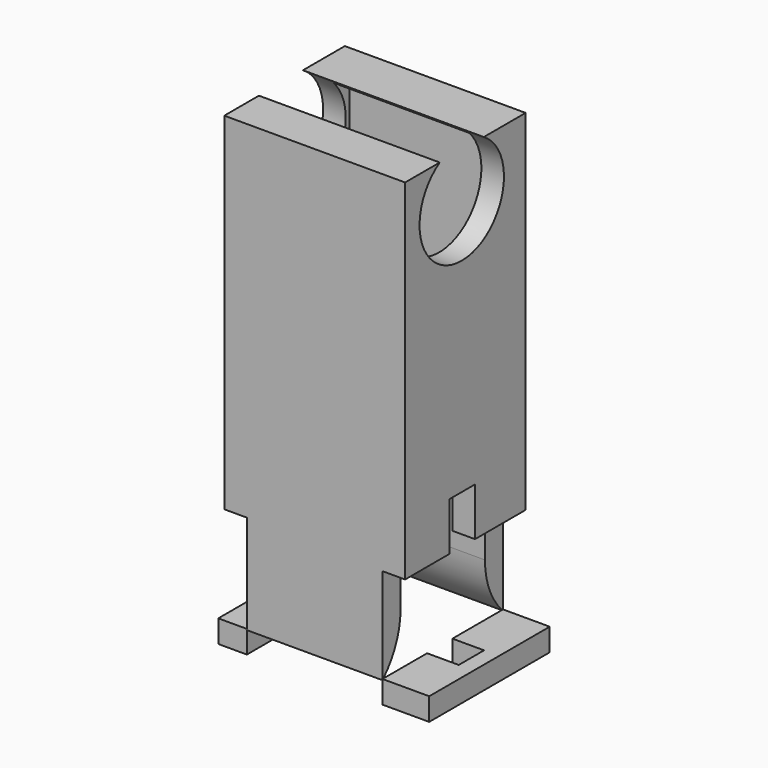
from build123d import *

# Parameters (mm, degrees)
F0_W         = 14
F0_H         = 10
F1_DEPTH     = 1.5
F2_W         = 9
F2_H         = 7
F3_DEPTH     = 25
F4_W         = 12
F4_H         = 10
F4_W_2       = 9
F4_H_2       = 7
F5_DEPTH     = 29
F6_W         = 12
F6_H         = 10
F7_DEPTH     = 0.5
F8_R         = 3.5
F9_DEPTH     = 25
F10_W        = 2.1
F10_H        = 2.1
F11_DEPTH    = 11
F12_W        = 10
F12_H        = 6.5
F13_DEPTH    = 1.5
F14_W        = 10
F14_H        = 6.3
F15_DEPTH    = 1.5
F16_T1_DEPTH = 9


# Not quite as in the source:
# - a fillet or chamfer that OpenCascade refuses, or shapes differently, is made with other operations: its cross-section is extruded or revolved along the edge and cut away or added


with BuildPart() as f1:
    # F0 (on Top) → F1 (new body)
    with BuildSketch(Plane.XY):
        with Locations((7, 5)):
            Rectangle(F0_W, F0_H)
    extrude(amount=F1_DEPTH)

    # F2 (on face) → F3 (cut)
    with BuildSketch(Plane.XY.offset(1.5)):
        with Locations((6.4, 5)):
            Rectangle(F2_W, F2_H)
    extrude(amount=-F3_DEPTH, mode=Mode.SUBTRACT)

    # F4 (on face) → F5 (join)
    with BuildSketch(Plane.XY.offset(1.5)):
        with Locations((6.4, 5)):
            Rectangle(F4_W, F4_H)
        with Locations((6.4, 5)):
            Rectangle(F4_W_2, F4_H_2, mode=Mode.SUBTRACT)
    extrude(amount=F5_DEPTH)

    # F6 (on face) → F7 (join)
    with BuildSketch(Plane.XY.offset(30.5)):
        with Locations((6.4, 5)):
            Rectangle(F6_W, F6_H)
    extrude(amount=F7_DEPTH)

    # F8 (on face) → F9 (cut)
    with BuildSketch(Plane.YZ.offset(12.4)):
        with Locations((4.7, 28.0150376887)):
            Circle(F8_R)
    extrude(amount=-F9_DEPTH, mode=Mode.SUBTRACT)

    # F10 (on face) → F11 (cut)
    with BuildSketch(Plane(origin=(0, 0, 0), x_dir=(1, 0, 0), z_dir=(0, 0, -1))):
        with Locations((11.95, -4.75)):
            Rectangle(F10_W, F10_H)
    extrude(amount=-F11_DEPTH, mode=Mode.SUBTRACT)

    # F12 (on face) → F13 (cut)
    with BuildSketch(Plane(origin=(0.4, 0, 0), x_dir=(0, -1, 0), z_dir=(-1, 0, 0))):
        with Locations((-5, 4.75)):
            Rectangle(F12_W, F12_H)
    extrude(amount=-F13_DEPTH, mode=Mode.SUBTRACT)

    # F14 (on face) → F15 (cut)
    with BuildSketch(Plane.YZ.offset(12.4)):
        with Locations((5, 4.65)):
            Rectangle(F14_W, F14_H)
    extrude(amount=-F15_DEPTH, mode=Mode.SUBTRACT)

    # F16: fillet of radius 5 on 2 edges, made by hand

    # F16_s2 → F16_t1 (cut)
    with BuildSketch(Plane.YZ.offset(1.9)):
        with BuildLine():
            ThreePointArc((8.5, 5), (9.9644660941, 1.4644660941), (13.5, 0))
            Line((13.5, 0), (13.5, -0.1))
            Line((13.5, -0.1), (8.4, -0.1))
            Line((8.4, -0.1), (8.4, 5))
            Line((8.4, 5), (8.5, 5))
        make_face()
        with BuildLine():
            ThreePointArc((1.5, 5), (0.0355339059, 1.4644660941), (-3.5, 0))
            Line((-3.5, 0), (-3.5, -0.1))
            Line((-3.5, -0.1), (1.6, -0.1))
            Line((1.6, -0.1), (1.6, 5))
            Line((1.6, 5), (1.5, 5))
        make_face()
    extrude(amount=F16_T1_DEPTH, mode=Mode.SUBTRACT)


solid = f1.part
